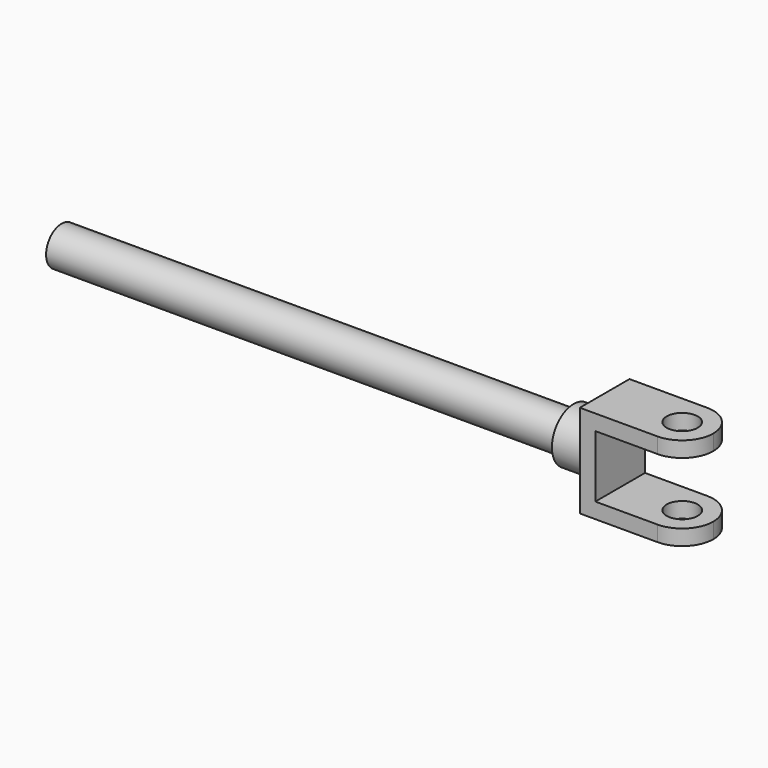
from build123d import *

# Parameters (mm, degrees)
F1_DEPTH = 6.35
F2_R     = 3.17499
F4_D     = 3.175
F5_R     = 2.778125
F6_DEPTH = 3.175
F7_R     = 1.984375
F8_DEPTH = 52.3875


# Not quite as in the source:
# - a fillet or chamfer is up to 0.001 mm smaller than in the source, because OpenCascade refuses the exact size


with BuildPart() as f1:
    # F0 (on Front) → F1 (new body)
    with BuildSketch(Plane.XZ):
        Polygon((33.251190576, 26.4741850346), (33.251190576, 28.0616850346), (22.138690576, 28.0616850346), (22.138690576, 18.5366850346), (33.251190576, 18.5366850346), (33.251190576, 20.1241850346), (23.726190576, 20.1241850346), (23.726190576, 26.4741850346), align=None)
    extrude(amount=F1_DEPTH)

    # F2 (radius 3.175 in the source; OpenCascade refuses exactly that, so slightly less here)
    f2_edges = [f1.edges().sort_by_distance(p)[0] for p in [
        (33.251191, -6.35, 19.330435),
        (33.251191, -6.35, 27.267935),
        (33.251191, 0, 27.267935),
        (33.251191, 0, 19.330435),
    ]]
    fillet(f2_edges, radius=F2_R)

    # F4 (through all)
    with Locations(Plane.XY.offset(28.0616850346)):
        with Locations((30.076190576, -3.175)):
            Hole(F4_D / 2)

    # F5 (on face) → F6 (join)
    with BuildSketch(Plane(origin=(22.138690576, 0, 0), x_dir=(0, -1, 0), z_dir=(-1, 0, 0))):
        with Locations((3.175, 23.2991850346)):
            Circle(F5_R)
    extrude(amount=F6_DEPTH)

    # F7 (on face) → F8 (join)
    with BuildSketch(Plane(origin=(18.963690576, 0, 0), x_dir=(0, -1, 0), z_dir=(-1, 0, 0))):
        with Locations((3.175, 23.2991850346)):
            Circle(F7_R)
    extrude(amount=F8_DEPTH)


solid = f1.part
